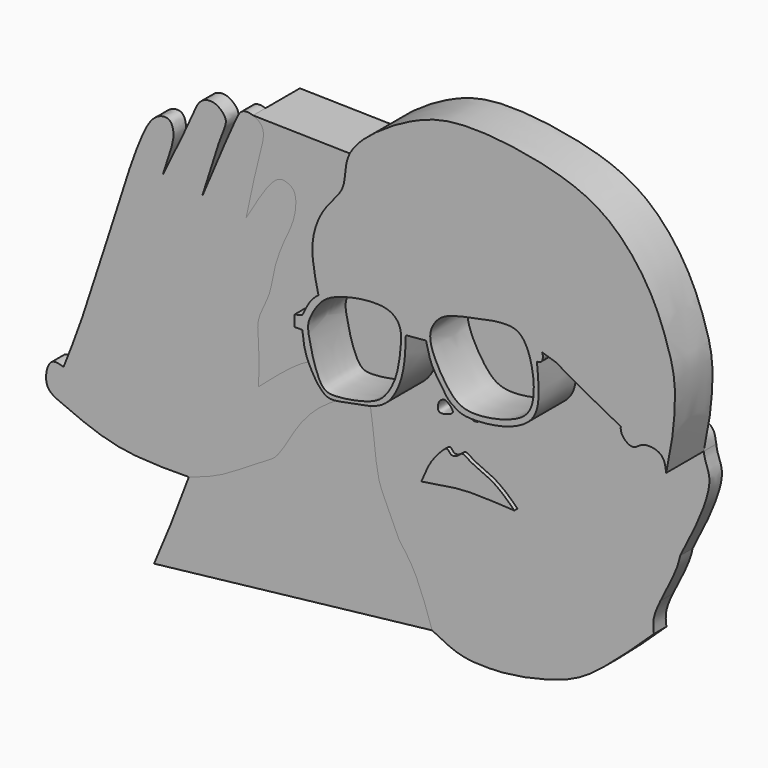
from build123d import *

# Parameters (mm, degrees)
F1_DEPTH = 2.032
F2_DEPTH = 7.62
F3_DEPTH = 6.096
F4_DEPTH = 0.508


with BuildPart() as f1:
    # F0 (on Front) → F1 (new body)
    with BuildSketch(Plane.XZ):
        with BuildLine():
            add(Edge.make_bspline(
                [(-55.2724488775, 1.5980589758), (-55.0387666607, 1.4893276605), (-53.1610247068, 0.7037993693), (-47.645902183, -1.7914382773), (-41.5273851628, -1.7336388853), (-38.236875087, -1.7025546404)],
                knots=[0.4025773763, 0.4025773763, 0.4025773763, 0.4025773763, 0.4429286296, 0.7004096007, 1, 1, 1, 1], degree=3))
            add(Edge.make_bspline(
                [(-38.236875087, -1.7025546404), (-36.8470247817, -1.2578424109), (-33.8979955842, -0.3142376614), (-28.947713113, 3.1761442834), (-26.6041221667, 4.0710783432), (-24.1821914599, 9.050699274), (-20.6594007368, 12.540658322), (-16.9473385578, 14.2485714757), (-19.5235868156, 17.3230254604), (-22.7338222113, 16.8764839895), (-26.3763270128, 14.0261410454), (-28.2677336447, 12.3693210091), (-29.1658081114, 11.5826325491)],
                knots=[0, 0, 0, 0, 0.1082269587, 0.2296394511, 0.3080097518, 0.422202912, 0.5383523625, 0.6262387345, 0.7089336404, 0.795556192, 0.9029263403, 1, 1, 1, 1], degree=3))
            add(Edge.make_bspline(
                [(-29.1658081114, 11.5826325491), (-29.1206047403, 13.2998509529), (-29.0754013691, 15.0170693567), (-29.1658081114, 16.4036750793)],
                knots=[0, 0, 0, 0, 0.1158770159, 0.1158770159, 0.1158770159, 0.1158770159], degree=3))
            add(Edge.make_bspline(
                [(-29.1658081114, 16.4036750793), (-29.2356020944, 17.474134358), (-29.5498842247, 19.2966582903), (-27.5955710546, 22.3999338138), (-27.3053052802, 25.4942442916), (-25.9984454014, 29.200289733), (-24.4043540317, 32.043761561), (-24.148458642, 35.4083621707), (-25.3526491591, 36.1725682292), (-26.6124513516, 36.4381295064), (-28.379316191, 34.4916214325), (-29.8928805536, 31.8989225999), (-30.7938195765, 30.3556360304)],
                knots=[0.1158770159, 0.1158770159, 0.1158770159, 0.1158770159, 0.2053340438, 0.3025428364, 0.3962351443, 0.4996270261, 0.5977233471, 0.6893356221, 0.7469512595, 0.8014595332, 0.8818201204, 1, 1, 1, 1], degree=3))
            add(Edge.make_bspline(
                [(-30.7938195765, 30.3556360304), (-30.5201103591, 31.7369642813), (-29.9644429575, 34.5412508423), (-28.7603523754, 38.8777185922), (-28.3063261099, 41.4426899651), (-29.3786765665, 42.211103985), (-29.8928805536, 42.3954501748)],
                knots=[0, 0, 0, 0, 0.1632749791, 0.3314706908, 0.4511843927, 0.5498826065, 0.5498826065, 0.5498826065, 0.5498826065], degree=3))
            add(Edge.make_bspline(
                [(-29.8928805536, 42.3954501748), (-30.3605475887, 42.5631124998), (-31.3900957362, 42.6319766993), (-32.350512941, 40.8561378233), (-34.7706749515, 35.0995445682), (-36.5325771272, 30.9086870402)],
                knots=[0.5498826065, 0.5498826065, 0.5498826065, 0.5498826065, 0.6396483458, 0.7376603877, 1, 1, 1, 1], degree=3))
            add(Edge.make_bspline(
                [(-36.5325771272, 30.9086870402), (-35.5904467123, 33.9733642825), (-34.1902283595, 38.5281660934), (-33.1565622295, 40.6384194548), (-33.9853152352, 41.6855732607), (-35.0402613991, 42.3581453136), (-36.9045620215, 42.133695175), (-38.147753948, 38.8294271181), (-40.2941233744, 34.4745690967), (-41.6216477752, 31.7810997367)],
                knots=[0, 0, 0, 0, 0.2346802659, 0.3487878218, 0.4337633641, 0.5234981812, 0.6226476014, 0.7666084362, 1, 1, 1, 1], degree=3))
            add(Edge.make_bspline(
                [(-41.6216477752, 31.7810997367), (-41.0515283232, 33.4498439856), (-40.175980835, 36.0125785679), (-40.2119720605, 37.3857844795), (-40.7080441223, 38.6665521664), (-42.8874872669, 38.3576530847), (-44.8034665439, 34.5769193652), (-47.3077170007, 27.0076271192), (-51.8383590008, 12.37570139), (-53.7422362276, 7.5605299543), (-54.5139610767, 5.6087300181)],
                knots=[0, 0, 0, 0, 0.1253598283, 0.1925183967, 0.2533503065, 0.3280194835, 0.4417189651, 0.6115587753, 0.842547754, 1, 1, 1, 1], degree=3))
            add(Edge.make_bspline(
                [(-54.5139610767, 5.6087300181), (-55.1115493055, 5.7886967446), (-56.4907744333, 6.2040573883), (-56.9600468727, 3.7434786677), (-56.6754974425, 2.8868434019)],
                knots=[0, 0, 0, 0, 0.1230929198, 0.2840967071, 0.2840967071, 0.2840967071, 0.2840967071], degree=3))
            add(Edge.make_bspline(
                [(-56.6754974425, 2.8868434019), (-56.4705322186, 2.2697961674), (-55.9799399318, 1.9318031129), (-55.3157672983, 1.6183563137)],
                knots=[0.2840967071, 0.2840967071, 0.2840967071, 0.2840967071, 0.4000701508, 0.4000701508, 0.4000701508, 0.4000701508], degree=3))
            add(Edge.make_bspline(
                [(-55.3157672983, 1.6183563137), (-55.3043199363, 1.6271325437), (-55.288226095, 1.6129308149), (-55.2724488775, 1.5980589758)],
                knots=[0.9660338474, 0.9660338474, 0.9660338474, 0.9660338474, 1, 1, 1, 1], degree=3))
        make_face()
    extrude(amount=-F1_DEPTH)


with BuildPart() as f1b:
    # F0 (on Front) → F1, piece 2 (new body)
    with BuildSketch(Plane.XZ):
        with BuildLine():
            add(Edge.make_bspline(
                [(-10.9039330855, 0), (-11.4311645648, 1.1654894447), (-12.3952525861, 3.2966869486), (-13.6285530402, 5.7883442969), (-14.0388844285, 9.2869362372), (-14.9210050461, 17.0677596487), (-15.1707846671, 17.3272378743)],
                knots=[0, 0, 0, 0, 0.2232565302, 0.4082437314, 0.6498522078, 0.970145573, 0.970145573, 0.970145573, 0.970145573], degree=3))
            add(Edge.make_bspline(
                [(-10.9039330855, 0), (-10.1947185931, -0.9460936084), (-8.5708818153, -3.1122952488), (-7.3173806659, -6.858217796), (-6.6113490611, -8.9680999517)],
                knots=[0, 0, 0, 0, 0.4367523276, 1, 1, 1, 1], degree=3))
            add(Edge.make_bspline(
                [(-6.6113490611, -8.9680999517), (-5.3664810433, -9.6084950105), (-3.0521274536, -10.7990634739), (0.0974631267, -10.9033388714), (3.5149397109, -10.8958044596), (11.1317982981, -9.2783327432), (15.5653502782, -6.1915067361), (20.7779108925, -1.3977852147), (21.8474367621, -0.3578969172), (22.2155340016, 0)],
                knots=[0, 0, 0, 0, 0.1358277735, 0.2525195367, 0.3786324058, 0.5641986285, 0.7292822553, 0.9068274482, 1, 1, 1, 1], degree=3))
            add(Edge.make_bspline(
                [(22.2155340016, 0), (22.1432270663, 0.5819174533), (22.0026611464, 1.7131749446), (22.6818828908, 3.2730999612), (23.0705857318, 4.0668730272)],
                knots=[0, 0, 0, 0, 0.2119085292, 0.4119538085, 0.4119538085, 0.4119538085, 0.4119538085], degree=3))
            add(Edge.make_bspline(
                [(23.0705857318, 4.0668730272), (23.263283306, 4.4603822278), (24.0920324831, 6.0702403182), (25.2751074501, 8.4805886248), (25.5248605365, 9.6102670006), (25.6226006895, 10.0523633882)],
                knots=[0.4119538085, 0.4119538085, 0.4119538085, 0.4119538085, 0.5111252988, 0.8086802899, 1, 1, 1, 1], degree=3))
            add(Edge.make_bspline(
                [(25.6226006895, 10.0523633882), (26.3408334739, 11.4332255528), (27.8263335133, 14.289222723), (29.99816716, 19.8869442748), (28.8924255609, 21.7349696727), (28.7443104073, 22.7239018185), (28.7032071532, 23.01570238)],
                knots=[0, 0, 0, 0, 0.0626684924, 0.1296154255, 0.1718989066, 0.19007829, 0.19007829, 0.19007829, 0.19007829], degree=3))
            add(Edge.make_bspline(
                [(28.7032071532, 23.01570238), (28.6587120715, 23.3315822322), (28.5499371625, 24.1630437776), (27.9112001442, 25.2996659751), (25.4950088973, 25.5423652371), (24.4215004111, 24.1195383258), (23.0363563605, 25.165011289), (22.8232023657, 25.8402836832), (22.8001871077, 25.9885722479)],
                knots=[0.19007829, 0.19007829, 0.19007829, 0.19007829, 0.2097578304, 0.2429662773, 0.283850236, 0.3177123001, 0.3542337069, 0.364538165, 0.364538165, 0.364538165, 0.364538165], degree=3))
            add(Edge.make_bspline(
                [(12.5391045585, 30.5677223951), (12.9953752774, 30.547227893), (14.543321963, 30.4772492354), (19.3876717143, 27.8456813073), (22.8001871077, 25.9885722479)],
                knots=[0, 0, 0, 0, 0.2946903168, 1, 1, 1, 1], degree=3))
            add(Edge.make_bspline(
                [(11.8854586035, 30.2835293114), (12.1413622821, 30.3135723453), (12.3972659607, 30.3436153792), (12.5391045585, 30.5677223951)],
                knots=[0, 0, 0, 0, 0.0708252116, 0.0708252116, 0.0708252116, 0.0708252116], degree=3))
            add(Edge.make_bspline(
                [(1.1116634123, 21.6421559453), (1.4237972027, 21.4316499302), (2.2422576345, 20.8796723831), (5.6264191324, 20.9494631201), (9.3347447125, 21.8172929341), (12.4966707544, 24.1810544555), (12.1073708827, 28.0679089218), (11.8854586035, 30.2835293114)],
                knots=[0, 0, 0, 0, 0.1213799954, 0.3182760936, 0.5345524296, 0.734681312, 1, 1, 1, 1], degree=3))
            add(Edge.make_bspline(
                [(-2.528490033, 28.0015207827), (-2.3254785693, 27.1323995558), (-1.938517827, 25.4757650539), (-0.7119782488, 23.7691926879), (0.2386305768, 22.2013159318), (0.8506711192, 21.8093162641), (1.1116634123, 21.6421559453)],
                knots=[0, 0, 0, 0, 0.2981463701, 0.5682976644, 0.8159092827, 1, 1, 1, 1], degree=3))
            add(Edge.make_bspline(
                [(-5.1545836031, 27.7654677629), (-4.2792190798, 27.8441521029), (-3.4038545564, 27.9228364428), (-2.528490033, 28.0015207827)],
                knots=[0, 0, 0, 0, 2.6366813359, 2.6366813359, 2.6366813359, 2.6366813359], degree=3))
            add(Edge.make_bspline(
                [(-15.1707846671, 17.3272378743), (-14.3986122925, 17.1507963987), (-12.0609527098, 17.8206353559), (-9.7131582596, 18.0416309659), (-7.4318253977, 19.0843558099), (-5.9261470855, 21.6285585172), (-5.2469620929, 24.5710791311), (-5.1856617571, 26.6908052329), (-5.1545836031, 27.7654677629)],
                knots=[0.380089275, 0.380089275, 0.380089275, 0.380089275, 0.4876812944, 0.5850173679, 0.6790122675, 0.7827370606, 0.8898516464, 1, 1, 1, 1], degree=3))
        make_face()
        with BuildLine():
            add(Edge.make_bspline(
                [(-7.605579216, 7.9525178298), (-6.2975526786, 8.1825504478), (-3.8643107516, 8.6104660861), (-1.0145520364, 8.8204355355), (1.7147537521, 8.7019483854), (3.5594020749, 8.6085931324), (4.4892118312, 8.5615366697)],
                knots=[0, 0, 0, 0, 0.2816917204, 0.5240139133, 0.760075402, 1, 1, 1, 1], degree=3))
            add(Edge.make_bspline(
                [(-7.605579216, 7.9525178298), (-7.2433932091, 8.8464607735), (-6.5546643194, 10.5463727506), (-5.0747224939, 12.2314557528), (-4.1606351561, 13.0378424569), (-3.8053357967, 12.0315840381), (-2.7854384192, 12.400138792), (-2.2611316959, 13.1051274552), (-1.1699659406, 12.1020410105), (1.9044487364, 11.1007282586), (3.6096506521, 9.4255904596), (4.4892118312, 8.5615366697)],
                knots=[0, 0, 0, 0, 0.1463115598, 0.2782244378, 0.3581635009, 0.4300398843, 0.5121124909, 0.5846970815, 0.6777570316, 0.8337836695, 1, 1, 1, 1], degree=3))
        make_face(mode=Mode.SUBTRACT)
        with BuildLine():
            add(Edge.make_bspline(
                [(-5.7602701709, 16.4020899683), (-5.5674825092, 16.18351098), (-4.696555253, 16.3614138349), (-3.4742240833, 16.8435024835), (-4.7353847706, 17.9643377195), (-5.1795569084, 17.9479564451), (-5.8383770068, 17.5753280539), (-5.953157379, 16.6207818204), (-5.7602701709, 16.4020899683)],
                knots=[0, 0, 0, 0, 0.1830897713, 0.355093566, 0.5521911405, 0.6696555206, 0.8168156898, 1, 1, 1, 1], degree=3))
        make_face(mode=Mode.SUBTRACT)
        with BuildLine():
            add(Edge.make_bspline(
                [(-1.5354838688, 16.9848185033), (-1.2983083887, 16.7120960081), (-0.5869849499, 16.7227972747), (0.0937505174, 17.4631145638), (0.212106106, 18.5672472651), (-1.029138043, 19.1387678545), (-2.054825103, 18.9340002703), (-1.8702060806, 17.3697076864), (-1.5354838688, 16.9848185033)],
                knots=[0, 0, 0, 0, 0.1521787911, 0.3096194464, 0.4649009807, 0.6420454688, 0.7852323456, 1, 1, 1, 1], degree=3))
        make_face(mode=Mode.SUBTRACT)
    extrude(amount=-F1_DEPTH)


with BuildPart() as f1c:
    # F0 (on Front) → F1, piece 3 (new body)
    with BuildSketch(Plane.XZ):
        with BuildLine():
            add(Edge.make_bspline(
                [(12.5106852502, 31.5908193588), (12.3064402033, 31.7978233371), (11.2467111567, 31.4606097042), (9.8518624239, 34.0807467832), (6.0643582494, 33.9469141756), (2.3794542405, 33.0855290488), (-1.3088887194, 32.749451576), (-2.1240387821, 30.5504436173), (-2.528490033, 29.4593665749)],
                knots=[0.1556963619, 0.1556963619, 0.1556963619, 0.1556963619, 0.2404363337, 0.3724355005, 0.5290856928, 0.697051941, 0.8496869141, 1, 1, 1, 1], degree=3))
            add(Edge.make_bspline(
                [(12.5106852502, 31.5908193588), (13.387351221, 31.3285350342), (14.723408881, 30.9288418811), (15.1807142816, 30.3932682155), (19.4372880907, 28.1587262513), (22.7937813016, 26.3952698884)],
                knots=[0, 0, 0, 0, 0.287019596, 0.4373090055, 1, 1, 1, 1], degree=3))
            add(Edge.make_bspline(
                [(22.7937813016, 26.3952698884), (22.8156224271, 26.5805502041), (23.0129515347, 27.2366706442), (24.1021137364, 28.2799243158), (23.3858815658, 33.1883702229), (17.995599049, 38.4159487026), (12.4352826838, 43.9765983444), (4.8791903274, 45.1635090529), (-0.0378177294, 44.7884802582), (-5.5452723549, 42.5538783771), (-11.0389478958, 37.1760956029), (-13.2939259106, 32.1707512568), (-14.4509887323, 29.6024344862)],
                knots=[0.3740429391, 0.3740429391, 0.3740429391, 0.3740429391, 0.3872440558, 0.4223577083, 0.4805187152, 0.5580271231, 0.6370626447, 0.7127070237, 0.774757023, 0.8417354125, 0.9187920818, 1, 1, 1, 1], degree=3))
            add(Edge.make_bspline(
                [(-5.3502218798, 29.2176697403), (-5.7347405428, 29.6046092529), (-6.5151306235, 30.3899125075), (-8.0814195647, 31.1783853328), (-12.7239869625, 30.1520839402), (-14.4509887323, 29.6024344862)],
                knots=[0, 0, 0, 0, 0.1349070048, 0.2737970832, 0.5476862699, 0.5476862699, 0.5476862699, 0.5476862699], degree=3))
            add(Edge.make_bspline(
                [(-2.528490033, 29.4593665749), (-3.4690673153, 29.3788009634), (-4.4096445975, 29.2982353518), (-5.3502218798, 29.2176697403)],
                knots=[0, 0, 0, 0, 2.8320642604, 2.8320642604, 2.8320642604, 2.8320642604], degree=3))
        make_face()
    extrude(amount=-F1_DEPTH)

    # F0 (on Front) → F3 (join)
    with BuildSketch(Plane.XZ):
        with BuildLine():
            add(Edge.make_bspline(
                [(-15.1707846671, 17.3272378743), (-15.1862660393, 17.3433203671), (-15.2007753347, 17.3433616813), (-15.2149589399, 17.3380284639)],
                knots=[0.970145573, 0.970145573, 0.970145573, 0.970145573, 0.9899973958, 0.9899973958, 0.9899973958, 0.9899973958], degree=3))
            add(Edge.make_bspline(
                [(-15.1707846671, 17.3272378743), (-14.3986122925, 17.1507963987), (-12.0609527098, 17.8206353559), (-9.7131582596, 18.0416309659), (-7.4318253977, 19.0843558099), (-5.9261470855, 21.6285585172), (-5.2469620929, 24.5710791311), (-5.1856617571, 26.6908052329), (-5.1545836031, 27.7654677629)],
                knots=[0.380089275, 0.380089275, 0.380089275, 0.380089275, 0.4876812944, 0.5850173679, 0.6790122675, 0.7827370606, 0.8898516464, 1, 1, 1, 1], degree=3))
            add(Edge.make_bspline(
                [(-5.1545836031, 27.7654677629), (-4.2792190798, 27.8441521029), (-3.4038545564, 27.9228364428), (-2.528490033, 28.0015207827)],
                knots=[0, 0, 0, 0, 2.6366813359, 2.6366813359, 2.6366813359, 2.6366813359], degree=3))
            add(Edge.make_bspline(
                [(-2.528490033, 28.0015207827), (-2.3254785693, 27.1323995558), (-1.938517827, 25.4757650539), (-0.7119782488, 23.7691926879), (0.2386305768, 22.2013159318), (0.8506711192, 21.8093162641), (1.1116634123, 21.6421559453)],
                knots=[0, 0, 0, 0, 0.2981463701, 0.5682976644, 0.8159092827, 1, 1, 1, 1], degree=3))
            add(Edge.make_bspline(
                [(1.1116634123, 21.6421559453), (1.4237972027, 21.4316499302), (2.2422576345, 20.8796723831), (5.6264191324, 20.9494631201), (9.3347447125, 21.8172929341), (12.4966707544, 24.1810544555), (12.1073708827, 28.0679089218), (11.8854586035, 30.2835293114)],
                knots=[0, 0, 0, 0, 0.1213799954, 0.3182760936, 0.5345524296, 0.734681312, 1, 1, 1, 1], degree=3))
            add(Edge.make_bspline(
                [(11.8854586035, 30.2835293114), (12.1413622821, 30.3135723453), (12.3972659607, 30.3436153792), (12.5391045585, 30.5677223951)],
                knots=[0, 0, 0, 0, 0.0708252116, 0.0708252116, 0.0708252116, 0.0708252116], degree=3))
            add(Edge.make_bspline(
                [(12.5391045585, 30.5677223951), (12.7090723521, 30.8362739429), (12.7152464708, 31.3834949359), (12.5106852502, 31.5908193588)],
                knots=[0.0708252116, 0.0708252116, 0.0708252116, 0.0708252116, 0.1556963619, 0.1556963619, 0.1556963619, 0.1556963619], degree=3))
            add(Edge.make_bspline(
                [(12.5106852502, 31.5908193588), (12.3064402033, 31.7978233371), (11.2467111567, 31.4606097042), (9.8518624239, 34.0807467832), (6.0643582494, 33.9469141756), (2.3794542405, 33.0855290488), (-1.3088887194, 32.749451576), (-2.1240387821, 30.5504436173), (-2.528490033, 29.4593665749)],
                knots=[0.1556963619, 0.1556963619, 0.1556963619, 0.1556963619, 0.2404363337, 0.3724355005, 0.5290856928, 0.697051941, 0.8496869141, 1, 1, 1, 1], degree=3))
            add(Edge.make_bspline(
                [(-2.528490033, 29.4593665749), (-3.4690673153, 29.3788009634), (-4.4096445975, 29.2982353518), (-5.3502218798, 29.2176697403)],
                knots=[0, 0, 0, 0, 2.8320642604, 2.8320642604, 2.8320642604, 2.8320642604], degree=3))
            add(Edge.make_bspline(
                [(-5.3502218798, 29.2176697403), (-5.7347405428, 29.6046092529), (-6.5151306235, 30.3899125075), (-8.0814195647, 31.1783853328), (-12.7239869625, 30.1520839402), (-14.4509887323, 29.6024344862)],
                knots=[0, 0, 0, 0, 0.1349070048, 0.2737970832, 0.5476862699, 0.5476862699, 0.5476862699, 0.5476862699], degree=3))
            add(Edge.make_bspline(
                [(-14.4509887323, 29.6024344862), (-15.4736908275, 29.2769411033), (-16.0217611566, 28.9975015656), (-16.5088865906, 28.6423619837)],
                knots=[0.5476862699, 0.5476862699, 0.5476862699, 0.5476862699, 0.7098789497, 0.7098789497, 0.7098789497, 0.7098789497], degree=3))
            add(Edge.make_bspline(
                [(-16.5088865906, 28.6423619837), (-16.9078254756, 28.3515149472), (-17.6898884514, 27.6053670225), (-18.2845526097, 26.3628008718), (-18.6069533229, 25.6891362369)],
                knots=[0.7098789497, 0.7098789497, 0.7098789497, 0.7098789497, 0.8427091457, 1, 1, 1, 1], degree=3))
            add(Edge.make_bspline(
                [(-18.6069533229, 25.6891362369), (-18.9525646468, 25.5951949706), (-19.2981759707, 25.5012537042), (-19.6437872946, 25.4073124379)],
                knots=[0, 0, 0, 0, 1.0744530416, 1.0744530416, 1.0744530416, 1.0744530416], degree=3))
            add(Edge.make_bspline(
                [(-19.6437872946, 25.4073124379), (-19.6437872946, 24.9371106426), (-19.6437872946, 24.4669088473), (-19.6437872946, 23.996707052)],
                knots=[0, 0, 0, 0, 1.4106053859, 1.4106053859, 1.4106053859, 1.4106053859], degree=3))
            add(Edge.make_bspline(
                [(-19.6437872946, 23.996707052), (-19.2981759707, 23.996707052), (-18.9525646468, 23.996707052), (-18.6069533229, 23.996707052)],
                knots=[0, 0, 0, 0, 1.0368339717, 1.0368339717, 1.0368339717, 1.0368339717], degree=3))
            add(Edge.make_bspline(
                [(-18.6069533229, 23.996707052), (-18.5412374364, 23.3794200199), (-18.4085187636, 22.1327577594), (-17.8063740332, 20.3760202119), (-16.7743550826, 18.6321715726), (-16.2278071772, 18.0427794664), (-15.6841109428, 17.4601064274), (-15.2149589399, 17.3380284639)],
                knots=[0, 0, 0, 0, 0.0837956623, 0.1692322766, 0.2554224195, 0.311137651, 0.3780141303, 0.3780141303, 0.3780141303, 0.3780141303], degree=3))
        make_face()
        with BuildLine():
            add(Edge.make_bspline(
                [(-17.7741199732, 23.7019918859), (-17.9000040169, 24.4785749381), (-17.876244843, 25.3444073375), (-16.53145708, 27.8224127085), (-14.3619247051, 29.5155606159), (-7.6787330026, 30.727185578), (-5.6368384035, 28.5735845405), (-5.803068546, 25.9507246984), (-6.2428063852, 22.5400940999), (-7.7029790138, 19.9127425636), (-9.5209866656, 18.4937712004), (-14.5119341523, 17.572187416), (-16.5181179601, 18.2376983892), (-17.5523314435, 22.3337707179), (-17.7741199732, 23.7019918859)],
                knots=[0, 0, 0, 0, 0.0616463908, 0.1357860661, 0.2160333731, 0.3353452776, 0.4084518795, 0.4825192301, 0.5708565879, 0.6503932483, 0.7222810325, 0.826126132, 0.8913884399, 1, 1, 1, 1], degree=3))
        make_face(mode=Mode.SUBTRACT)
        with BuildLine():
            add(Edge.make_bspline(
                [(-1.981225796, 28.7297666073), (-2.0099583439, 27.8659764626), (-1.2245361199, 25.8038161404), (0.5560774902, 22.986913942), (2.7896708281, 21.2226336575), (8.5013480904, 22.2131397933), (11.6807087758, 24.3122910872), (11.4920003535, 29.3107413325), (10.3443170094, 32.3663721727), (8.438041624, 33.6532837617), (3.2410685101, 32.5220801663), (0.0182153578, 31.8083955798), (-1.40005037, 30.599353336), (-1.9581636056, 29.4230880942), (-1.981225796, 28.7297666073)],
                knots=[0, 0, 0, 0, 0.0799525882, 0.1647615246, 0.2398387116, 0.3487837737, 0.4358562514, 0.5356486778, 0.6184896405, 0.6833640143, 0.7895554099, 0.8752560947, 0.9358260248, 1, 1, 1, 1], degree=3))
        make_face(mode=Mode.SUBTRACT)
        with BuildLine():
            add(Edge.make_bspline(
                [(12.5106852502, 31.5908193588), (12.3064402033, 31.7978233371), (11.2467111567, 31.4606097042), (9.8518624239, 34.0807467832), (6.0643582494, 33.9469141756), (2.3794542405, 33.0855290488), (-1.3088887194, 32.749451576), (-2.1240387821, 30.5504436173), (-2.528490033, 29.4593665749)],
                knots=[0.1556963619, 0.1556963619, 0.1556963619, 0.1556963619, 0.2404363337, 0.3724355005, 0.5290856928, 0.697051941, 0.8496869141, 1, 1, 1, 1], degree=3))
            add(Edge.make_bspline(
                [(12.5106852502, 31.5908193588), (13.387351221, 31.3285350342), (14.723408881, 30.9288418811), (15.1807142816, 30.3932682155), (19.4372880907, 28.1587262513), (22.7937813016, 26.3952698884)],
                knots=[0, 0, 0, 0, 0.287019596, 0.4373090055, 1, 1, 1, 1], degree=3))
            add(Edge.make_bspline(
                [(22.7937813016, 26.3952698884), (22.8156224271, 26.5805502041), (23.0129515347, 27.2366706442), (24.1021137364, 28.2799243158), (23.3858815658, 33.1883702229), (17.995599049, 38.4159487026), (12.4352826838, 43.9765983444), (4.8791903274, 45.1635090529), (-0.0378177294, 44.7884802582), (-5.5452723549, 42.5538783771), (-11.0389478958, 37.1760956029), (-13.2939259106, 32.1707512568), (-14.4509887323, 29.6024344862)],
                knots=[0.3740429391, 0.3740429391, 0.3740429391, 0.3740429391, 0.3872440558, 0.4223577083, 0.4805187152, 0.5580271231, 0.6370626447, 0.7127070237, 0.774757023, 0.8417354125, 0.9187920818, 1, 1, 1, 1], degree=3))
            add(Edge.make_bspline(
                [(-5.3502218798, 29.2176697403), (-5.7347405428, 29.6046092529), (-6.5151306235, 30.3899125075), (-8.0814195647, 31.1783853328), (-12.7239869625, 30.1520839402), (-14.4509887323, 29.6024344862)],
                knots=[0, 0, 0, 0, 0.1349070048, 0.2737970832, 0.5476862699, 0.5476862699, 0.5476862699, 0.5476862699], degree=3))
            add(Edge.make_bspline(
                [(-2.528490033, 29.4593665749), (-3.4690673153, 29.3788009634), (-4.4096445975, 29.2982353518), (-5.3502218798, 29.2176697403)],
                knots=[0, 0, 0, 0, 2.8320642604, 2.8320642604, 2.8320642604, 2.8320642604], degree=3))
        make_face()
        with BuildLine():
            add(Edge.make_bspline(
                [(28.7032071532, 23.01570238), (28.6587120715, 23.3315822322), (28.5499371625, 24.1630437776), (27.9112001442, 25.2996659751), (25.4950088973, 25.5423652371), (24.4215004111, 24.1195383258), (23.0363563605, 25.165011289), (22.8232023657, 25.8402836832), (22.8001871077, 25.9885722479)],
                knots=[0.19007829, 0.19007829, 0.19007829, 0.19007829, 0.2097578304, 0.2429662773, 0.283850236, 0.3177123001, 0.3542337069, 0.364538165, 0.364538165, 0.364538165, 0.364538165], degree=3))
            add(Edge.make_bspline(
                [(28.7032071532, 23.01570238), (29.0733638248, 24.882575143), (29.8037584238, 28.5475704943), (29.9588887399, 34.020370016), (28.8959372711, 37.7482572166), (26.8921444274, 43.2967602737), (21.5300055701, 50.2301331364), (13.2060581543, 53.4493931882), (2.0165960728, 54.7630837167), (-3.8705835572, 52.9962280774), (-9.2948279348, 49.8120638694), (-13.3076224029, 45.9762793506), (-12.9477095519, 43.1118508118), (-13.345126994, 42.0467145741)],
                knots=[0, 0, 0, 0, 0.0704590805, 0.1383236595, 0.1955605255, 0.2662451799, 0.351644913, 0.4399912623, 0.537690659, 0.6102025565, 0.6837476464, 0.7507995529, 0.80694987, 0.80694987, 0.80694987, 0.80694987], degree=3))
            add(Edge.make_bspline(
                [(-13.345126994, 42.0467145741), (-13.7455741567, 40.9734582467), (-15.8334977626, 39.1894448843), (-17.8474025405, 34.4108172054), (-16.9683293303, 30.6223719124), (-16.5088865906, 28.6423619837)],
                knots=[0.80694987, 0.80694987, 0.80694987, 0.80694987, 0.8635282503, 0.928673186, 1, 1, 1, 1], degree=3))
            add(Edge.make_bspline(
                [(-14.4509887323, 29.6024344862), (-15.4736908275, 29.2769411033), (-16.0217611566, 28.9975015656), (-16.5088865906, 28.6423619837)],
                knots=[0.5476862699, 0.5476862699, 0.5476862699, 0.5476862699, 0.7098789497, 0.7098789497, 0.7098789497, 0.7098789497], degree=3))
            add(Edge.make_bspline(
                [(22.7937813016, 26.3952698884), (22.8156224271, 26.5805502041), (23.0129515347, 27.2366706442), (24.1021137364, 28.2799243158), (23.3858815658, 33.1883702229), (17.995599049, 38.4159487026), (12.4352826838, 43.9765983444), (4.8791903274, 45.1635090529), (-0.0378177294, 44.7884802582), (-5.5452723549, 42.5538783771), (-11.0389478958, 37.1760956029), (-13.2939259106, 32.1707512568), (-14.4509887323, 29.6024344862)],
                knots=[0.3740429391, 0.3740429391, 0.3740429391, 0.3740429391, 0.3872440558, 0.4223577083, 0.4805187152, 0.5580271231, 0.6370626447, 0.7127070237, 0.774757023, 0.8417354125, 0.9187920818, 1, 1, 1, 1], degree=3))
            add(Edge.make_bspline(
                [(22.8001871077, 25.9885722479), (22.7789579635, 26.125352784), (22.7780557408, 26.2618684821), (22.7937813016, 26.3952698884)],
                knots=[0.364538165, 0.364538165, 0.364538165, 0.364538165, 0.3740429391, 0.3740429391, 0.3740429391, 0.3740429391], degree=3))
        make_face()
    extrude(amount=F3_DEPTH)


with BuildPart() as f1d:
    # F0 (on Front) → F1, piece 4 (new body)
    with BuildSketch(Plane.XZ):
        with BuildLine():
            add(Edge.make_bspline(
                [(-1.981225796, 28.7297666073), (-2.0099583439, 27.8659764626), (-1.2245361199, 25.8038161404), (0.5560774902, 22.986913942), (2.7896708281, 21.2226336575), (8.5013480904, 22.2131397933), (11.6807087758, 24.3122910872), (11.4920003535, 29.3107413325), (10.3443170094, 32.3663721727), (8.438041624, 33.6532837617), (3.2410685101, 32.5220801663), (0.0182153578, 31.8083955798), (-1.40005037, 30.599353336), (-1.9581636056, 29.4230880942), (-1.981225796, 28.7297666073)],
                knots=[0, 0, 0, 0, 0.0799525882, 0.1647615246, 0.2398387116, 0.3487837737, 0.4358562514, 0.5356486778, 0.6184896405, 0.6833640143, 0.7895554099, 0.8752560947, 0.9358260248, 1, 1, 1, 1], degree=3))
        make_face()
        with BuildLine():
            add(Edge.make_bspline(
                [(1.3580559753, 26.5756584704), (1.3111418804, 26.2677605346), (2.3529672917, 26.4951156491), (3.6595665009, 26.7553726216)],
                knots=[0, 0, 0, 0, 0.1705292223, 0.1705292223, 0.1705292223, 0.1705292223], degree=3))
            add(Edge.make_bspline(
                [(3.3064371795, 28.1224267366), (2.4276997732, 27.6421593346), (1.4025792094, 26.8678651501), (1.3580559753, 26.5756584704)],
                knots=[0.8381613774, 0.8381613774, 0.8381613774, 0.8381613774, 1, 1, 1, 1], degree=3))
            add(Edge.make_bspline(
                [(5.4770470597, 28.2232537866), (4.8458204698, 28.4206595505), (4.5820040206, 28.736882239), (3.5913468891, 28.278142022), (3.3064371795, 28.1224267366)],
                knots=[0.6452933564, 0.6452933564, 0.6452933564, 0.6452933564, 0.7856890522, 0.8381613774, 0.8381613774, 0.8381613774, 0.8381613774], degree=3))
            add(Edge.make_bspline(
                [(5.2064743743, 27.0371501369), (6.9000151167, 27.3018232782), (10.0845010041, 27.4996620119), (6.3873680405, 27.938565829), (5.4770470597, 28.2232537866)],
                knots=[0.234836749, 0.234836749, 0.234836749, 0.234836749, 0.4428222476, 0.6452933564, 0.6452933564, 0.6452933564, 0.6452933564], degree=3))
            add(Edge.make_bspline(
                [(3.6595665009, 26.7553726216), (4.0564422175, 26.8344249214), (4.5794965557, 26.9363380208), (5.1046124366, 27.0212307566), (5.2064743743, 27.0371501369)],
                knots=[0.1705292223, 0.1705292223, 0.1705292223, 0.1705292223, 0.2223269785, 0.234836749, 0.234836749, 0.234836749, 0.234836749], degree=3))
        make_face(mode=Mode.SUBTRACT)
        with BuildLine():
            add(Edge.make_bspline(
                [(3.3064371795, 28.1224267366), (3.2901646966, 27.9179758444), (3.2583069716, 27.474182034), (3.517319707, 27.0192514892), (3.6595665009, 26.7553726216)],
                knots=[0, 0, 0, 0, 0.4652023668, 1, 1, 1, 1], degree=3))
            add(Edge.make_bspline(
                [(3.6595665009, 26.7553726216), (4.0564422175, 26.8344249214), (4.5794965557, 26.9363380208), (5.1046124366, 27.0212307566), (5.2064743743, 27.0371501369)],
                knots=[0.1705292223, 0.1705292223, 0.1705292223, 0.1705292223, 0.2223269785, 0.234836749, 0.234836749, 0.234836749, 0.234836749], degree=3))
            add(Edge.make_bspline(
                [(5.4770470597, 28.2232537866), (5.4960314615, 28.0249458642), (5.5441354044, 27.6108732146), (5.3135265911, 27.2574859086), (5.2064743743, 27.0371501369)],
                knots=[0, 0, 0, 0, 0.4854878277, 1, 1, 1, 1], degree=3))
            add(Edge.make_bspline(
                [(5.4770470597, 28.2232537866), (4.8458204698, 28.4206595505), (4.5820040206, 28.736882239), (3.5913468891, 28.278142022), (3.3064371795, 28.1224267366)],
                knots=[0.6452933564, 0.6452933564, 0.6452933564, 0.6452933564, 0.7856890522, 0.8381613774, 0.8381613774, 0.8381613774, 0.8381613774], degree=3))
        make_face()
        with BuildLine():
            add(Edge.make_bspline(
                [(3.3064371795, 28.1224267366), (2.4276997732, 27.6421593346), (1.4025792094, 26.8678651501), (1.3580559753, 26.5756584704)],
                knots=[0.8381613774, 0.8381613774, 0.8381613774, 0.8381613774, 1, 1, 1, 1], degree=3))
            add(Edge.make_bspline(
                [(1.3580559753, 26.5756584704), (1.3111418804, 26.2677605346), (2.3529672917, 26.4951156491), (3.6595665009, 26.7553726216)],
                knots=[0, 0, 0, 0, 0.1705292223, 0.1705292223, 0.1705292223, 0.1705292223], degree=3))
            add(Edge.make_bspline(
                [(3.3064371795, 28.1224267366), (3.2901646966, 27.9179758444), (3.2583069716, 27.474182034), (3.517319707, 27.0192514892), (3.6595665009, 26.7553726216)],
                knots=[0, 0, 0, 0, 0.4652023668, 1, 1, 1, 1], degree=3))
        make_face()
        with BuildLine():
            add(Edge.make_bspline(
                [(5.4770470597, 28.2232537866), (5.4960314615, 28.0249458642), (5.5441354044, 27.6108732146), (5.3135265911, 27.2574859086), (5.2064743743, 27.0371501369)],
                knots=[0, 0, 0, 0, 0.4854878277, 1, 1, 1, 1], degree=3))
            add(Edge.make_bspline(
                [(5.2064743743, 27.0371501369), (6.9000151167, 27.3018232782), (10.0845010041, 27.4996620119), (6.3873680405, 27.938565829), (5.4770470597, 28.2232537866)],
                knots=[0.234836749, 0.234836749, 0.234836749, 0.234836749, 0.4428222476, 0.6452933564, 0.6452933564, 0.6452933564, 0.6452933564], degree=3))
        make_face()
    extrude(amount=-F1_DEPTH)


with BuildPart() as f1e:
    # F0 (on Front) → F1, piece 5 (new body)
    with BuildSketch(Plane.XZ):
        with BuildLine():
            add(Edge.make_bspline(
                [(-17.7741199732, 23.7019918859), (-17.9000040169, 24.4785749381), (-17.876244843, 25.3444073375), (-16.53145708, 27.8224127085), (-14.3619247051, 29.5155606159), (-7.6787330026, 30.727185578), (-5.6368384035, 28.5735845405), (-5.803068546, 25.9507246984), (-6.2428063852, 22.5400940999), (-7.7029790138, 19.9127425636), (-9.5209866656, 18.4937712004), (-14.5119341523, 17.572187416), (-16.5181179601, 18.2376983892), (-17.5523314435, 22.3337707179), (-17.7741199732, 23.7019918859)],
                knots=[0, 0, 0, 0, 0.0616463908, 0.1357860661, 0.2160333731, 0.3353452776, 0.4084518795, 0.4825192301, 0.5708565879, 0.6503932483, 0.7222810325, 0.826126132, 0.8913884399, 1, 1, 1, 1], degree=3))
        make_face()
        with BuildLine():
            add(Edge.make_bspline(
                [(-11.5092201158, 23.7019918859), (-10.9328729895, 23.6377568404), (-10.3565258633, 23.5735217949), (-9.692972526, 23.7019918859)],
                knots=[0, 0, 0, 0, 0.4314434241, 0.4314434241, 0.4314434241, 0.4314434241], degree=3))
            add(Edge.make_bspline(
                [(-11.5092201158, 23.7019918859), (-11.1664199478, 24.0826609893), (-10.8236197797, 24.4633300928), (-10.5674620718, 24.7446522117)],
                knots=[0, 0, 0, 0, 0.2206888001, 0.2206888001, 0.2206888001, 0.2206888001], degree=3))
            add(Edge.make_bspline(
                [(-10.5674620718, 24.7446522117), (-10.3908856673, 24.9385751221), (-10.0900870319, 25.2644976523), (-9.2886477601, 25.3726536708), (-8.467935109, 25.4378504326), (-8.1441280449, 25.4307262207)],
                knots=[0.2206888001, 0.2206888001, 0.2206888001, 0.2206888001, 0.3728155315, 0.5586309077, 0.6854927968, 0.6854927968, 0.6854927968, 0.6854927968], degree=3))
            add(Edge.make_bspline(
                [(-8.1441280449, 25.4307262207), (-7.8269941619, 25.4237488282), (-7.1472872358, 25.3373681509), (-6.7638914296, 24.9468623633), (-6.7667942494, 24.8791892081)],
                knots=[0.6854927968, 0.6854927968, 0.6854927968, 0.6854927968, 0.8097402515, 0.9593942358, 0.9593942358, 0.9593942358, 0.9593942358], degree=3))
            add(Edge.make_bspline(
                [(-8.2981174025, 24.1602344814), (-7.8005912251, 24.3713472356), (-7.2836927372, 24.6252682219), (-6.7667942494, 24.8791892081)],
                knots=[0.7135260529, 0.7135260529, 0.7135260529, 0.7135260529, 1, 1, 1, 1], degree=3))
            add(Edge.make_bspline(
                [(-9.692972526, 23.7019918859), (-9.25913379, 23.7859870959), (-8.788017072, 23.9523578445), (-8.2981174025, 24.1602344814)],
                knots=[0.4314434241, 0.4314434241, 0.4314434241, 0.4314434241, 0.7135260529, 0.7135260529, 0.7135260529, 0.7135260529], degree=3))
        make_face(mode=Mode.SUBTRACT)
        with BuildLine():
            add(Edge.make_bspline(
                [(-10.5674620718, 24.7446522117), (-10.3908856673, 24.9385751221), (-10.0900870319, 25.2644976523), (-9.2886477601, 25.3726536708), (-8.467935109, 25.4378504326), (-8.1441280449, 25.4307262207)],
                knots=[0.2206888001, 0.2206888001, 0.2206888001, 0.2206888001, 0.3728155315, 0.5586309077, 0.6854927968, 0.6854927968, 0.6854927968, 0.6854927968], degree=3))
            add(Edge.make_bspline(
                [(-10.5674620718, 24.7446522117), (-10.5021159378, 24.5271979366), (-10.3673915001, 24.078871415), (-9.9222200319, 23.8301002212), (-9.692972526, 23.7019918859)],
                knots=[0, 0, 0, 0, 0.4850354923, 1, 1, 1, 1], degree=3))
            add(Edge.make_bspline(
                [(-9.692972526, 23.7019918859), (-9.25913379, 23.7859870959), (-8.788017072, 23.9523578445), (-8.2981174025, 24.1602344814)],
                knots=[0.4314434241, 0.4314434241, 0.4314434241, 0.4314434241, 0.7135260529, 0.7135260529, 0.7135260529, 0.7135260529], degree=3))
            add(Edge.make_bspline(
                [(-8.1441280449, 25.4307262207), (-8.1507378428, 25.2541725209), (-8.1676198267, 24.8711644077), (-8.2499130911, 24.4034039905), (-8.2981174025, 24.1602344814)],
                knots=[0, 0, 0, 0, 0.4655446921, 1, 1, 1, 1], degree=3))
        make_face()
        with BuildLine():
            add(Edge.make_bspline(
                [(-8.1441280449, 25.4307262207), (-7.8269941619, 25.4237488282), (-7.1472872358, 25.3373681509), (-6.7638914296, 24.9468623633), (-6.7667942494, 24.8791892081)],
                knots=[0.6854927968, 0.6854927968, 0.6854927968, 0.6854927968, 0.8097402515, 0.9593942358, 0.9593942358, 0.9593942358, 0.9593942358], degree=3))
            add(Edge.make_bspline(
                [(-8.1441280449, 25.4307262207), (-8.1507378428, 25.2541725209), (-8.1676198267, 24.8711644077), (-8.2499130911, 24.4034039905), (-8.2981174025, 24.1602344814)],
                knots=[0, 0, 0, 0, 0.4655446921, 1, 1, 1, 1], degree=3))
            add(Edge.make_bspline(
                [(-8.2981174025, 24.1602344814), (-7.8005912251, 24.3713472356), (-7.2836927372, 24.6252682219), (-6.7667942494, 24.8791892081)],
                knots=[0.7135260529, 0.7135260529, 0.7135260529, 0.7135260529, 1, 1, 1, 1], degree=3))
        make_face()
        with BuildLine():
            add(Edge.make_bspline(
                [(-11.5092201158, 23.7019918859), (-11.1664199478, 24.0826609893), (-10.8236197797, 24.4633300928), (-10.5674620718, 24.7446522117)],
                knots=[0, 0, 0, 0, 0.2206888001, 0.2206888001, 0.2206888001, 0.2206888001], degree=3))
            add(Edge.make_bspline(
                [(-11.5092201158, 23.7019918859), (-10.9328729895, 23.6377568404), (-10.3565258633, 23.5735217949), (-9.692972526, 23.7019918859)],
                knots=[0, 0, 0, 0, 0.4314434241, 0.4314434241, 0.4314434241, 0.4314434241], degree=3))
            add(Edge.make_bspline(
                [(-10.5674620718, 24.7446522117), (-10.5021159378, 24.5271979366), (-10.3673915001, 24.078871415), (-9.9222200319, 23.8301002212), (-9.692972526, 23.7019918859)],
                knots=[0, 0, 0, 0, 0.4850354923, 1, 1, 1, 1], degree=3))
        make_face()
    extrude(amount=-F1_DEPTH)


with BuildPart() as f2:
    # F0 (on Front) → F2 (new body)
    with BuildSketch(Plane.XZ):
        with BuildLine():
            add(Edge.make_bspline(
                [(-10.9039330855, 0), (-10.1947185931, -0.9460936084), (-8.5708818153, -3.1122952488), (-7.3173806659, -6.858217796), (-6.6113490611, -8.9680999517)],
                knots=[0, 0, 0, 0, 0.4367523276, 1, 1, 1, 1], degree=3))
            add(Edge.make_bspline(
                [(-10.9039330855, 0), (-11.4311645648, 1.1654894447), (-12.3952525861, 3.2966869486), (-13.6285530402, 5.7883442969), (-14.0388844285, 9.2869362372), (-14.9210050461, 17.0677596487), (-15.1707846671, 17.3272378743)],
                knots=[0, 0, 0, 0, 0.2232565302, 0.4082437314, 0.6498522078, 0.970145573, 0.970145573, 0.970145573, 0.970145573], degree=3))
            add(Edge.make_bspline(
                [(-15.2149589399, 17.3380284639), (-15.2004013805, 17.3342404438), (-15.1856776811, 17.3306409297), (-15.1707846671, 17.3272378743)],
                knots=[0.3780141303, 0.3780141303, 0.3780141303, 0.3780141303, 0.380089275, 0.380089275, 0.380089275, 0.380089275], degree=3))
            add(Edge.make_bspline(
                [(-18.6069533229, 23.996707052), (-18.5412374364, 23.3794200199), (-18.4085187636, 22.1327577594), (-17.8063740332, 20.3760202119), (-16.7743550826, 18.6321715726), (-16.2278071772, 18.0427794664), (-15.6841109428, 17.4601064274), (-15.2149589399, 17.3380284639)],
                knots=[0, 0, 0, 0, 0.0837956623, 0.1692322766, 0.2554224195, 0.311137651, 0.3780141303, 0.3780141303, 0.3780141303, 0.3780141303], degree=3))
            add(Edge.make_bspline(
                [(-19.6437872946, 23.996707052), (-19.2981759707, 23.996707052), (-18.9525646468, 23.996707052), (-18.6069533229, 23.996707052)],
                knots=[0, 0, 0, 0, 1.0368339717, 1.0368339717, 1.0368339717, 1.0368339717], degree=3))
            add(Edge.make_bspline(
                [(-19.6437872946, 25.4073124379), (-19.6437872946, 24.9371106426), (-19.6437872946, 24.4669088473), (-19.6437872946, 23.996707052)],
                knots=[0, 0, 0, 0, 1.4106053859, 1.4106053859, 1.4106053859, 1.4106053859], degree=3))
            add(Edge.make_bspline(
                [(-18.6069533229, 25.6891362369), (-18.9525646468, 25.5951949706), (-19.2981759707, 25.5012537042), (-19.6437872946, 25.4073124379)],
                knots=[0, 0, 0, 0, 1.0744530416, 1.0744530416, 1.0744530416, 1.0744530416], degree=3))
            add(Edge.make_bspline(
                [(-16.5088865906, 28.6423619837), (-16.9078254756, 28.3515149472), (-17.6898884514, 27.6053670225), (-18.2845526097, 26.3628008718), (-18.6069533229, 25.6891362369)],
                knots=[0.7098789497, 0.7098789497, 0.7098789497, 0.7098789497, 0.8427091457, 1, 1, 1, 1], degree=3))
            add(Edge.make_bspline(
                [(-13.345126994, 42.0467145741), (-13.7455741567, 40.9734582467), (-15.8334977626, 39.1894448843), (-17.8474025405, 34.4108172054), (-16.9683293303, 30.6223719124), (-16.5088865906, 28.6423619837)],
                knots=[0.80694987, 0.80694987, 0.80694987, 0.80694987, 0.8635282503, 0.928673186, 1, 1, 1, 1], degree=3))
            add(Edge.make_bspline(
                [(-29.8928805536, 42.3954501748), (-24.3769627004, 42.2792049746), (-18.8610448472, 42.1629597743), (-13.345126994, 42.0467145741)],
                knots=[0, 0, 0, 0, 16.5514278656, 16.5514278656, 16.5514278656, 16.5514278656], degree=3))
            add(Edge.make_bspline(
                [(-30.7938195765, 30.3556360304), (-30.5201103591, 31.7369642813), (-29.9644429575, 34.5412508423), (-28.7603523754, 38.8777185922), (-28.3063261099, 41.4426899651), (-29.3786765665, 42.211103985), (-29.8928805536, 42.3954501748)],
                knots=[0, 0, 0, 0, 0.1632749791, 0.3314706908, 0.4511843927, 0.5498826065, 0.5498826065, 0.5498826065, 0.5498826065], degree=3))
            add(Edge.make_bspline(
                [(-29.1658081114, 16.4036750793), (-29.2356020944, 17.474134358), (-29.5498842247, 19.2966582903), (-27.5955710546, 22.3999338138), (-27.3053052802, 25.4942442916), (-25.9984454014, 29.200289733), (-24.4043540317, 32.043761561), (-24.148458642, 35.4083621707), (-25.3526491591, 36.1725682292), (-26.6124513516, 36.4381295064), (-28.379316191, 34.4916214325), (-29.8928805536, 31.8989225999), (-30.7938195765, 30.3556360304)],
                knots=[0.1158770159, 0.1158770159, 0.1158770159, 0.1158770159, 0.2053340438, 0.3025428364, 0.3962351443, 0.4996270261, 0.5977233471, 0.6893356221, 0.7469512595, 0.8014595332, 0.8818201204, 1, 1, 1, 1], degree=3))
            add(Edge.make_bspline(
                [(-29.1658081114, 11.5826325491), (-29.1206047403, 13.2998509529), (-29.0754013691, 15.0170693567), (-29.1658081114, 16.4036750793)],
                knots=[0, 0, 0, 0, 0.1158770159, 0.1158770159, 0.1158770159, 0.1158770159], degree=3))
            add(Edge.make_bspline(
                [(-38.236875087, -1.7025546404), (-36.8470247817, -1.2578424109), (-33.8979955842, -0.3142376614), (-28.947713113, 3.1761442834), (-26.6041221667, 4.0710783432), (-24.1821914599, 9.050699274), (-20.6594007368, 12.540658322), (-16.9473385578, 14.2485714757), (-19.5235868156, 17.3230254604), (-22.7338222113, 16.8764839895), (-26.3763270128, 14.0261410454), (-28.2677336447, 12.3693210091), (-29.1658081114, 11.5826325491)],
                knots=[0, 0, 0, 0, 0.1082269587, 0.2296394511, 0.3080097518, 0.422202912, 0.5383523625, 0.6262387345, 0.7089336404, 0.795556192, 0.9029263403, 1, 1, 1, 1], degree=3))
            add(Edge.make_bspline(
                [(-38.236875087, -1.7025546404), (-39.1175770599, -4.0574532729), (-40.733582511, -8.3784712159), (-42.1221540294, -11.6132661762), (-42.7539721131, -13.0851399153)],
                knots=[0, 0, 0, 0, 0.5449870062, 1, 1, 1, 1], degree=3))
            add(Edge.make_bspline(
                [(-42.7539721131, -13.0851399153), (-30.7064310958, -11.7127932608), (-18.6588900785, -10.3404466063), (-6.6113490611, -8.9680999517)],
                knots=[0, 0, 0, 0, 36.3763552207, 36.3763552207, 36.3763552207, 36.3763552207], degree=3))
        make_face()
    extrude(amount=-F2_DEPTH)


with BuildPart() as f4:
    # F0 (on Front) → F4 (new body)
    with BuildSketch(Plane.XZ):
        with BuildLine():
            add(Edge.make_bspline(
                [(-7.605579216, 7.9525178298), (-7.2433932091, 8.8464607735), (-6.5546643194, 10.5463727506), (-5.0747224939, 12.2314557528), (-4.1606351561, 13.0378424569), (-3.8053357967, 12.0315840381), (-2.7854384192, 12.400138792), (-2.2611316959, 13.1051274552), (-1.1699659406, 12.1020410105), (1.9044487364, 11.1007282586), (3.6096506521, 9.4255904596), (4.4892118312, 8.5615366697)],
                knots=[0, 0, 0, 0, 0.1463115598, 0.2782244378, 0.3581635009, 0.4300398843, 0.5121124909, 0.5846970815, 0.6777570316, 0.8337836695, 1, 1, 1, 1], degree=3))
            add(Edge.make_bspline(
                [(-7.605579216, 7.9525178298), (-6.9619343353, 8.8083899727), (-5.8479421343, 10.2896957681), (-4.1623440168, 9.5716638415), (-1.8702911323, 10.9258623063), (1.3721693128, 9.9004097021), (3.440134349, 9.0121502053), (4.4892118312, 8.5615366697)],
                knots=[0, 0, 0, 0, 0.204285367, 0.3535681124, 0.545595803, 0.7694810103, 1, 1, 1, 1], degree=3))
        make_face()
        with BuildLine():
            add(Edge.make_bspline(
                [(-7.605579216, 7.9525178298), (-6.9619343353, 8.8083899727), (-5.8479421343, 10.2896957681), (-4.1623440168, 9.5716638415), (-1.8702911323, 10.9258623063), (1.3721693128, 9.9004097021), (3.440134349, 9.0121502053), (4.4892118312, 8.5615366697)],
                knots=[0, 0, 0, 0, 0.204285367, 0.3535681124, 0.545595803, 0.7694810103, 1, 1, 1, 1], degree=3))
            add(Edge.make_bspline(
                [(-7.605579216, 7.9525178298), (-6.2975526786, 8.1825504478), (-3.8643107516, 8.6104660861), (-1.0145520364, 8.8204355355), (1.7147537521, 8.7019483854), (3.5594020749, 8.6085931324), (4.4892118312, 8.5615366697)],
                knots=[0, 0, 0, 0, 0.2816917204, 0.5240139133, 0.760075402, 1, 1, 1, 1], degree=3))
        make_face()
    extrude(amount=F4_DEPTH)


solid = Compound([f1.part, f1b.part, f1c.part, f1d.part, f1e.part, f2.part, f4.part])
